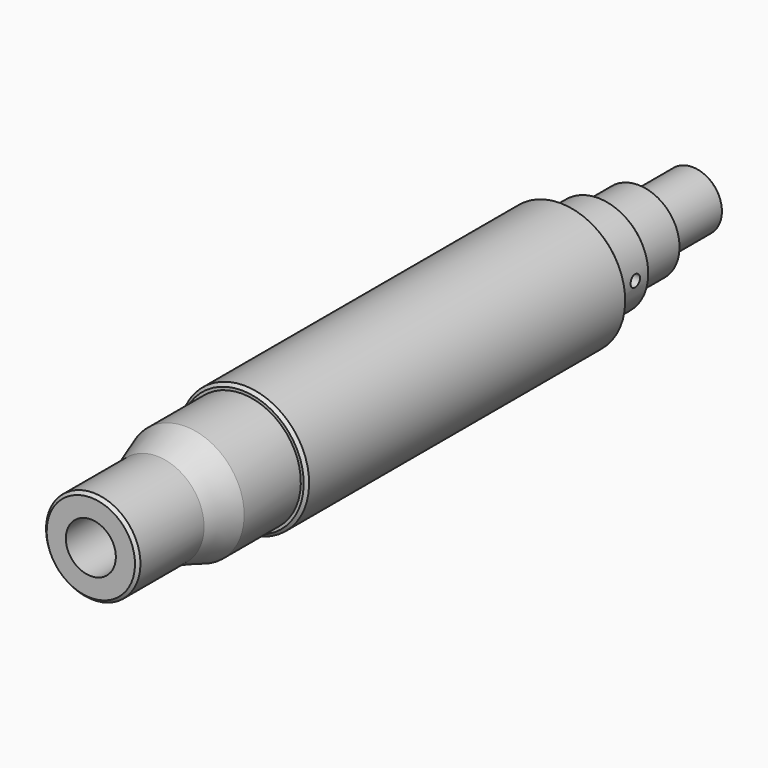
from build123d import *

# Parameters (mm, degrees)
F2_SIZE        = 0.8128
F5_D           = 8.4836
F5_DEPTH       = 63.5
F5_CSINK_D     = 9.525
F5_CSINK_ANGLE = 60
F5_TIP         = 2.5487305738
F7_D           = 3.175
F7_DEPTH       = 38.1
F7_TIP         = 0.9538662327


# Not quite as in the source:
# - a fillet or chamfer that OpenCascade refuses, or shapes differently, is made with other operations: its cross-section is extruded or revolved along the edge and cut away or added


with BuildPart() as f1:
    # F0 (on Right) → F1 (revolve)
    with BuildSketch(Plane.YZ):
        Polygon((-177.8, 0), (0, 0), (0, 7.9375), (-19.05, 7.9375), (-19.05, 11.1125), (-31.75, 11.1125), (-31.75, 13.5128), (-44.45, 13.5128), (-44.45, 17.4625), (-152.4, 17.4625), (-152.4, 15.875), (-171.45, 15.875), (-180.975, 12.7), (-203.2, 12.7), (-203.2, 6.731), (-177.8, 6.731), align=None)
    revolve(axis=Axis((0, -88.9, 0), (0, -1, 0)))

    # F2
    f2_edges = [f1.edges().sort_by_distance(p)[0] for p in [
        (0, -203.2, -12.7),
        (0, -152.4, -17.4625),
        (0, -44.45, -17.4625),
        (0, -31.75, -13.5128),
        (0, 0, -7.9375),
    ]]
    chamfer(f2_edges, length=F2_SIZE)

    # F3: fillet of radius 3.175 on 1 edges, made by hand

    # F3_s1 → F3_t2 (revolve)
    with BuildSketch(Plane.YZ):
        with BuildLine():
            ThreePointArc((-41.2742745857, 13.5124), (-43.5064480149, 14.4289646435), (-44.4503999697, 16.6496950798))
            Line((-44.4503999697, 16.6496950798), (-44.7680125081, 16.6457880193))
            ThreePointArc((-44.7680125081, 16.6457880193), (-44.7676365685, 15.0812475399), (-44.7676365685, 13.5128))
            Line((-44.7676365685, 13.5128), (-44.45, 13.1951634315))
            ThreePointArc((-44.45, 13.1951634315), (-42.8621372928, 13.1951634315), (-41.2742745857, 13.1947634315))
            Line((-41.2742745857, 13.1947634315), (-41.2742745857, 13.5124))
        make_face()
    revolve(axis=Axis((0, -44.45, 0), (0, -1, 0)))

    # F5
    with Locations(Plane(origin=(0, 0, 0), x_dir=(-1, 0, 0), z_dir=(0, 1, 0))):
        with Locations((0, 0)):
            CounterSinkHole(F5_D / 2, F5_CSINK_D / 2, depth=F5_DEPTH, counter_sink_angle=F5_CSINK_ANGLE)
            with Locations((0, 0, -(F5_DEPTH + F5_TIP / 2))):  # 118° drill point
                Cone(0, F5_D / 2, F5_TIP, mode=Mode.SUBTRACT)

    # F7 (one way)
    with BuildSketch(Plane(origin=(0, 0, 0), x_dir=(0, 1, 0), z_dir=(-1, 0, 0))):
        with Locations((-36.915011704, 0)):
            Circle(F7_D / 2)
    extrude(amount=-F7_DEPTH, mode=Mode.SUBTRACT)
    with Locations(Plane(origin=(0, 0, 0), x_dir=(0, 1, 0), z_dir=(-1, 0, 0))):
        with Locations((-36.915011704, 0)):
            with Locations((0, 0, -(F7_DEPTH + F7_TIP / 2))):  # 118° drill point
                Cone(0, F7_D / 2, F7_TIP, mode=Mode.SUBTRACT)


solid = f1.part
